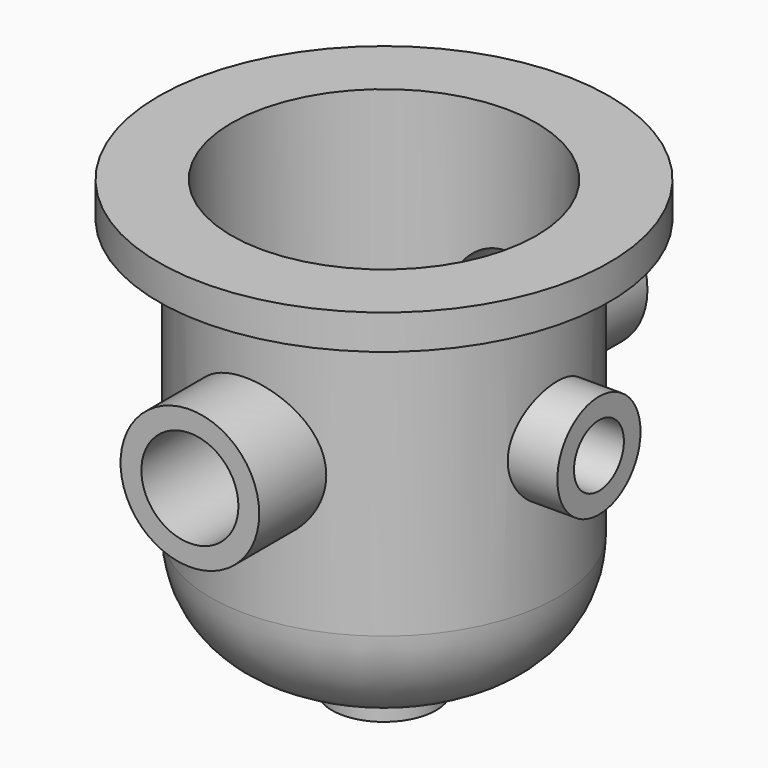
from build123d import *

# Parameters (mm, degrees)
F3_R      = 9.525
F4_DEPTH  = 6.35
F6_R      = 12.7
F8_R      = 8.89
F9_DEPTH  = 101.6
F10_R     = 5.715
F11_DEPTH = 25.4
F13_R     = 9.525
F15_R     = 5.715
F16_DEPTH = 25.4


# Not quite as in the source:
# - a pattern or mirror of a feature is missing from the dataset's text; its kind, count and spacing are read off the source's solid


with BuildPart() as f1:
    # F0 (on Front) → F1 (revolve)
    with BuildSketch(Plane.XZ):
        with BuildLine():
            Line((-27.94, 0), (-41.275, 0))
            Line((-41.275, 0), (-41.275, -6.35))
            Line((-41.275, -6.35), (-31.75, -6.35))
            Line((-31.75, -6.35), (-31.75, -57.15))
            ThreePointArc((-31.75, -57.15), (-26.1703841816, -70.6203841816), (-12.7, -76.2))
            Line((-12.7, -76.2), (0, -76.2))
            Line((0, -76.2), (0, -72.39))
            Line((0, -72.39), (-12.7, -72.39))
            ThreePointArc((-12.7, -72.39), (-23.4763073453, -67.9263073453), (-27.94, -57.15))
            Line((-27.94, -57.15), (-27.94, 0))
        make_face()
    revolve(axis=Axis((0, 0, -38.1), (0, 0, 1)))



with BuildPart() as f2:
    # F0 (on Front) → F2 (revolve)
    with BuildSketch(Plane.XZ):
        with BuildLine():
            Line((-27.94, 0), (-41.275, 0))
            Line((-41.275, 0), (-41.275, -6.35))
            Line((-41.275, -6.35), (-31.75, -6.35))
            Line((-31.75, -6.35), (-31.75, -57.15))
            ThreePointArc((-31.75, -57.15), (-26.1703841816, -70.6203841816), (-12.7, -76.2))
            Line((-12.7, -76.2), (0, -76.2))
            Line((0, -76.2), (0, -72.39))
            Line((0, -72.39), (-12.7, -72.39))
            ThreePointArc((-12.7, -72.39), (-23.4763073453, -67.9263073453), (-27.94, -57.15))
            Line((-27.94, -57.15), (-27.94, 0))
        make_face()
    revolve(axis=Axis((0, 0, -38.1), (0, 0, 1)))


with BuildPart() as f1_1:
    add(f1.part)

    add(f2.part)  # F4 merges F2
    # F3 (on face) → F4 (join)
    with BuildSketch(Plane(origin=(0, 0, -76.2), x_dir=(1, 0, 0), z_dir=(0, 0, -1))):
        Circle(F3_R)
    extrude(amount=F4_DEPTH)

    # F6 (on offset) → F7 (join, up to the next surface of F1)
    with BuildSketch(Plane.XZ.offset(44.45)):
        with Locations((0, -31.75)):
            Circle(F6_R)
    f7 = extrude(until=Until.NEXT, dir=(0, 1, 0))

    # F7_copies: F7 across plane
    add(f7.mirror(Plane.ZX))

    # F8 (on face) → F9 (cut)
    with BuildSketch(Plane.XZ.offset(44.45)):
        with Locations((0, -31.75)):
            Circle(F8_R)
    extrude(amount=-F9_DEPTH, mode=Mode.SUBTRACT)

    # F10 (on face) → F11 (cut)
    with BuildSketch(Plane(origin=(0, 0, -82.55), x_dir=(1, 0, 0), z_dir=(0, 0, -1))):
        Circle(F10_R)
    extrude(amount=-F11_DEPTH, mode=Mode.SUBTRACT)

    # F13 (on offset) → F14 (join, up to the next surface of F1)
    with BuildSketch(Plane.YZ.offset(39.37)):
        with Locations((0, -31.75)):
            Circle(F13_R)
    extrude(until=Until.NEXT, dir=(-1, 0, 0))

    # F15 (on face) → F16 (cut)
    with BuildSketch(Plane.YZ.offset(39.37)):
        with Locations((0, -31.75)):
            Circle(F15_R)
    extrude(amount=-F16_DEPTH, mode=Mode.SUBTRACT)


solid = f1_1.part
